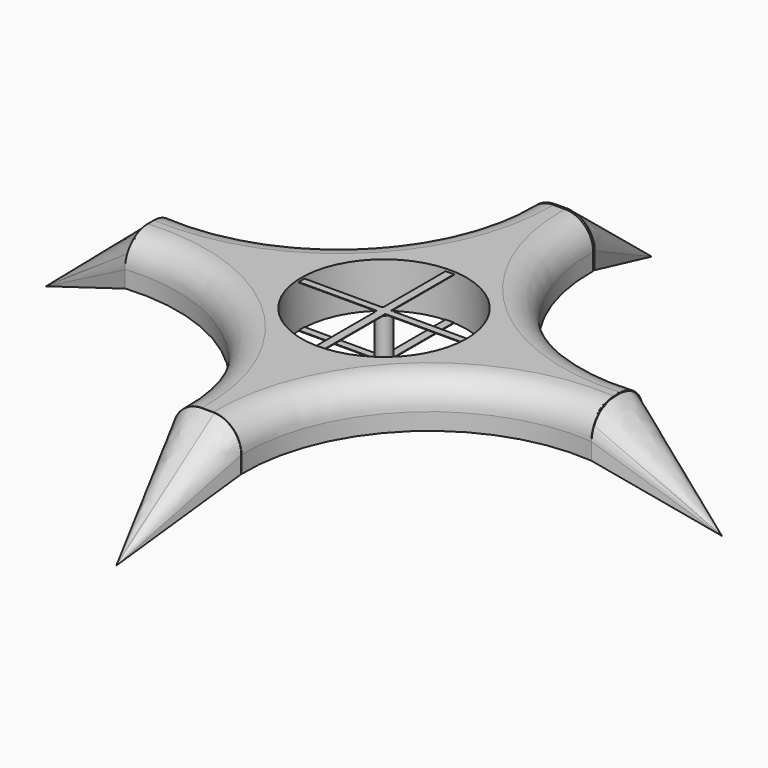
from build123d import *

# Parameters (mm, degrees)
F1_DEPTH       = 8
F5_R           = 5
F10_R          = 14.5809762942
F11_DEPTH      = 25
F11_DEPTH_BACK = 25
F17_R          = 1.3377868925
F18_DEPTH      = 7
F19_W          = 13.7937454856
F19_H          = 1.2778390591
F19_W_2        = 1.4747540699
F19_H_2        = 13.8842168999
F20_DEPTH      = 0.1
F21_W          = 13.7960873644
F21_H          = 1.2778390591
F21_W_2        = 1.4737510647
F21_H_2        = 13.8842168999
F22_DEPTH      = 0.1


# Not quite as in the source:
# - a feature names something its author has since deleted; it is built from what else it names


with BuildPart() as f1:
    # F0 (on Top) → F1 (new body)
    with BuildSketch(Plane.XY):
        with BuildLine():
            Line((-6, -38.9283647568), (0, -38.9283647568))
            Line((0, -38.9283647568), (0, 38.6506099872))
            Line((0, 38.6506099872), (-6, 38.6506099872))
            ThreePointArc((-6, 38.6506099872), (-16.2563291401, 14.3645411148), (-41.1563329399, 5.7045619305))
            Line((-41.1563329399, 5.7045619305), (-41.1563329399, -5.7045619305))
            ThreePointArc((-41.1563329399, -5.7045619305), (-16.1530460363, -14.4594456673), (-6, -38.9283647568))
        make_face()
        with BuildLine():
            Line((0, 38.6506099872), (0, -38.9283647568))
            Line((0, -38.9283647568), (6, -38.9283647568))
            ThreePointArc((6, -38.9283647568), (16.1530460363, -14.4594456673), (41.1563329399, -5.7045619305))
            Line((41.1563329399, -5.7045619305), (41.1563329399, 5.7045619305))
            ThreePointArc((41.1563329399, 5.7045619305), (16.2563291401, 14.3645411148), (6, 38.6506099872))
            Line((6, 38.6506099872), (0, 38.6506099872))
        make_face()
    extrude(amount=F1_DEPTH)

    # F5
    f5_edges = [f1.edges().sort_by_distance(p)[0] for p in [
        (-16.256329, 14.364541, 8),
        (-16.153046, -14.459446, 8),
        (16.256329, 14.364541, 8),
        (16.153046, -14.459446, 8),
    ]]
    fillet(f5_edges, radius=F5_R)

    # F10 (on Top) → F11 (cut, two sides)
    with BuildSketch(Plane.XY) as f11_sk:
        Circle(F10_R)
    extrude(amount=F11_DEPTH, mode=Mode.SUBTRACT)
    extrude(f11_sk.sketch, amount=-F11_DEPTH_BACK, mode=Mode.SUBTRACT)


with BuildPart() as f7:
    # F6 (on offset) → F7 section 0
    with BuildSketch(Plane.YZ.offset(41), mode=Mode.PRIVATE) as f7_s0:
        with BuildLine():
            Line((-5.6745633483, 2.9871875886), (-5.6745633483, 0))
            Line((-5.6745633483, 0), (5.680473987, 0))
            Line((5.680473987, 0), (5.680473987, 2.9871875886))
            add(Edge.make_bspline(
                [(5.680473987, 2.9871875886), (5.6961226516, 3.2023706582), (5.7266473384, 3.6221122778), (5.5095213329, 4.1705030453), (5.4189197792, 4.6854509336), (5.1653598653, 5.2792204603), (4.8671516526, 5.7675621219), (4.595492144, 6.1533733509), (4.1731740718, 6.5852177534), (3.6655723563, 7.0548230975), (2.9133413088, 7.5120975715), (2.0228145415, 7.8302873353), (1.3427473514, 7.9431760952), (0.7054569456, 8.0192411539), (-0.0052608695, 8.0094879795), (-0.6967338383, 7.9690324076), (-1.4140359274, 7.9528726283), (-1.9769670867, 7.8166335645), (-2.831114124, 7.5524617191), (-3.4441109512, 7.1858192873), (-3.8874893713, 6.884099922), (-4.2378609304, 6.5250253974), (-4.5111891113, 6.161764951), (-4.8527214432, 5.8131409825), (-5.022034993, 5.4567339521), (-5.1115825772, 5.2682352252)],
                knots=[0, 0, 0, 0, 0.0434863796, 0.0848256485, 0.1243592318, 0.1681716105, 0.2094747234, 0.2467932906, 0.2887889342, 0.3342469985, 0.3856749903, 0.4388627149, 0.4840956225, 0.5275602038, 0.5734684376, 0.6194034944, 0.6650441984, 0.7068937948, 0.7583696913, 0.8048710099, 0.8445998947, 0.882945876, 0.9196464802, 0.9575021397, 1, 1, 1, 1], degree=3))
            add(Edge.make_bspline(
                [(-5.1115825772, 5.2682352252), (-5.1876140748, 5.1405504387), (-5.3386246291, 4.8869483001), (-5.4298509883, 4.4603913926), (-5.6042277019, 4.0039908588), (-5.6752105609, 3.4265059116), (-5.6747687115, 3.1265850958), (-5.6745633483, 2.9871875886)],
                knots=[0, 0, 0, 0, 0.1927235014, 0.3827792915, 0.5867141249, 0.8079125632, 1, 1, 1, 1], degree=3))
        make_face()
    loft([Vertex(59.6456676722, 0, -8), f7_s0.sketch])


with BuildPart() as f9_1:
    # F9: instance of F7
    add(f7.part.mirror(Plane.YZ))


with BuildPart() as f15:
    # F13 (on offset) → F15 section 0
    with BuildSketch(Plane.XZ.offset(39), mode=Mode.PRIVATE) as f15_s0:
        with BuildLine():
            Line((-5.9944099137, 2.9958747894), (-5.9944099137, 0))
            Line((-5.9944099137, 0), (5.9937159531, 0))
            Line((5.9937159531, 0), (5.9937159531, 2.9904348776))
            add(Edge.make_bspline(
                [(1.2747923611, 7.9939775169), (1.4824839899, 7.9738728024), (1.9417054276, 7.9294198027), (2.9066530946, 7.6548688525), (3.4852965721, 7.3598152646), (4.1590321718, 6.8772754783), (4.6271761756, 6.4649031497), (5.123048457, 5.8613971166), (5.475565689, 5.2424580454), (5.6755920242, 4.8013575587), (5.892310974, 4.1137787102), (5.9984549521, 3.4762948253), (5.9952085186, 3.1434582903), (5.9937159531, 2.9904348776)],
                knots=[0, 0, 0, 0, 0.0901408322, 0.1993079971, 0.2897259787, 0.3881183325, 0.4758975639, 0.573044131, 0.6653592716, 0.7420254803, 0.835035104, 0.9241564892, 1, 1, 1, 1], degree=3))
            add(Edge.make_bspline(
                [(-5.9944099137, 2.9958747894), (-5.9950314515, 3.0479435495), (-5.9963679382, 3.1599064882), (-5.9858142016, 3.3813314), (-5.9646795578, 3.5305374515), (-5.9516586953, 3.7341965228), (-5.9018897214, 3.9408938339), (-5.8803328007, 4.1073797979), (-5.7960635617, 4.3768885226), (-5.74913918, 4.5723993195), (-5.6203314712, 4.9297471084), (-5.4836570267, 5.1988546444), (-5.4592090914, 5.270703893), (-5.3537695157, 5.4444498536), (-5.295526214, 5.5532759218), (-5.2180785314, 5.6862072163), (-5.0492178435, 5.9193146032), (-4.961360939, 6.0561793869), (-4.8747004771, 6.1501514649), (-4.7780479662, 6.2676655241), (-4.7121245787, 6.3575768778), (-4.4969781008, 6.5644294278), (-4.293631571, 6.7654278403), (-4.1636212216, 6.8683144457), (-3.9538061718, 7.0370130479), (-3.7360017211, 7.1784048192), (-3.6369210607, 7.2467137809), (-3.4014865011, 7.3869954226), (-3.2868331685, 7.4397869865), (-3.1681660923, 7.4993179406), (-3.0211153204, 7.5762029169), (-2.9250525886, 7.6095624185), (-2.5706425561, 7.7548356943), (-2.3335590973, 7.8169101439), (-1.8761051772, 7.923622144), (-1.6577938155, 7.9531586472), (-1.3119293852, 7.993050517), (-0.9738346206, 8.002401008), (0.326799832, 7.9975287536), (1.2747923611, 7.9939775169)],
                knots=[0, 0, 0, 0, 0.0225922841, 0.0485799646, 0.0703773601, 0.0953767047, 0.1208450417, 0.1439685284, 0.1728943558, 0.1983584542, 0.2331066781, 0.2631175547, 0.2787030186, 0.3031680151, 0.3230289605, 0.3447420766, 0.3747142758, 0.39730409, 0.4170698345, 0.4382806743, 0.4569453263, 0.4872616232, 0.5172585751, 0.5398068451, 0.5688071761, 0.5968393041, 0.6167877586, 0.645427363, 0.6655976282, 0.6857678614, 0.7078632653, 0.7261916835, 0.7595514909, 0.7890147822, 0.8262060834, 0.8534043783, 0.8844257561, 0.9157614812, 1, 1, 1, 1], degree=3))
        make_face()
    loft([Vertex(0, -59.0698996127, -8), f15_s0.sketch])


with BuildPart() as f16_1:
    # F16: instance of F15
    add(f15.part.mirror(Plane.XZ))


with BuildPart() as f18:
    # F17 (on offset) → F18 (new body)
    with BuildSketch(Plane.XY.offset(7.5)):
        Circle(F17_R)
    extrude(amount=-F18_DEPTH)

    # F19 (on offset) → F20 (join)
    with BuildSketch(Plane.XY.offset(7.5)):
        with Locations((7.6342497778, 0)):
            Rectangle(F19_W, F19_H)
        Rectangle(F19_W_2, F19_H)
        with Locations((0, 7.5810279795)):
            Rectangle(F19_W_2, F19_H_2)
        with Locations((-7.6342497778, 0)):
            Rectangle(F19_W, F19_H)
        with Locations((0, -7.5810279795)):
            Rectangle(F19_W_2, F19_H_2)
    extrude(amount=F20_DEPTH)


with BuildPart() as f22:
    # F21 (on Top) → F22 (new body)
    with BuildSketch(Plane.XY):
        with Locations((7.6360394938, -0.0199771021)):
            Rectangle(F21_W, F21_H)
        with Locations((0.0011202792, -0.0199771021)):
            Rectangle(F21_W_2, F21_H)
        with Locations((0.0011202792, 7.5610508775)):
            Rectangle(F21_W_2, F21_H_2)
        with Locations((-7.6337989354, -0.0199771021)):
            Rectangle(F21_W, F21_H)
        with Locations((0.0011202792, -7.6010050816)):
            Rectangle(F21_W_2, F21_H_2)
    extrude(amount=F22_DEPTH)


solid = Compound([f1.part, f7.part, f9_1.part, f15.part, f16_1.part, f18.part, f22.part])
